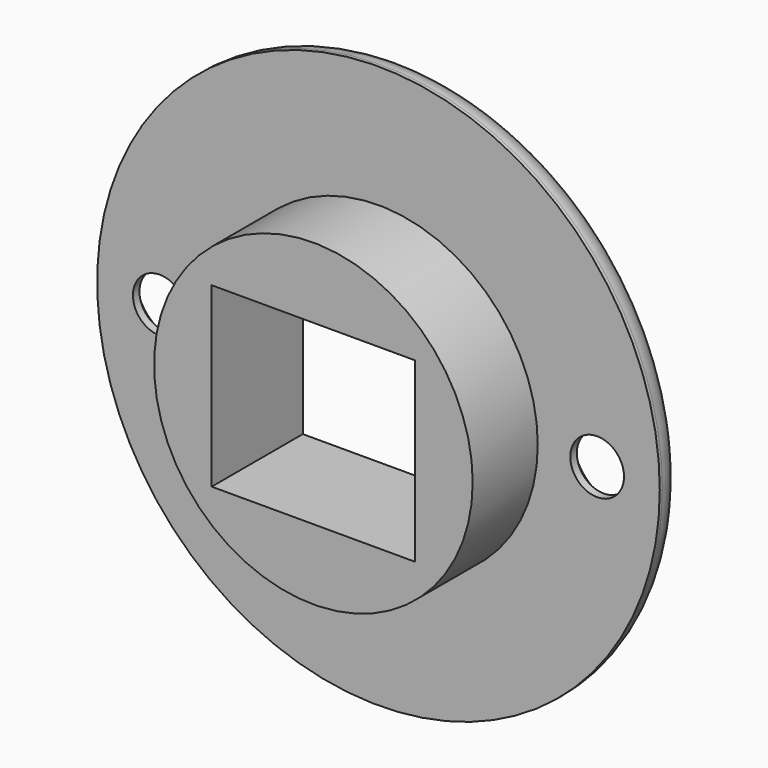
from build123d import *

# Parameters (mm, degrees)
F0_R     = 17.2924664606
F0_R_2   = 1.65
F0_R_3   = 9.7924664606
F1_DEPTH = 2
F2_DEPTH = 5
F3_SIZE  = 1.5


# Not quite as in the source:
# - a fillet or chamfer that OpenCascade refuses, or shapes differently, is made with other operations: its cross-section is extruded or revolved along the edge and cut away or added


with BuildPart() as f1:
    # F0 (on Front) → F1 (new body)
    with BuildSketch(Plane.XZ):
        Circle(F0_R)
        with Locations((-13.4424664606, 0)):
            Circle(F0_R_2, mode=Mode.SUBTRACT)
        Circle(F0_R_3, mode=Mode.SUBTRACT)
        with Locations((13.4424664606, 0)):
            Circle(F0_R_2, mode=Mode.SUBTRACT)
        Circle(F0_R_3)
        with BuildLine():
            ThreePointArc((8.2924664606, 0), (7.7650793743, -2.9100759974), (6.25, -5.45))
            ThreePointArc((6.25, -5.45), (0, -8.2924664606), (-6.25, -5.45))
            ThreePointArc((-6.25, -5.45), (-8.2924664606, 0), (-6.25, 5.45))
            ThreePointArc((-6.25, 5.45), (0, 8.2924664606), (6.25, 5.45))
            ThreePointArc((6.25, 5.45), (7.7650793743, 2.9100759974), (8.2924664606, 0))
        make_face(mode=Mode.SUBTRACT)
        with BuildLine():
            ThreePointArc((-6.25, 5.45), (-8.2924664606, 0), (-6.25, -5.45))
            Line((-6.25, -5.45), (-6.25, 5.45))
        make_face()
        with BuildLine():
            Line((-6.25, 5.45), (6.25, 5.45))
            ThreePointArc((6.25, 5.45), (0, 8.2924664606), (-6.25, 5.45))
        make_face()
        with BuildLine():
            Line((6.25, 5.45), (6.25, -5.45))
            ThreePointArc((6.25, -5.45), (7.7650793743, -2.9100759974), (8.2924664606, 0))
            ThreePointArc((8.2924664606, 0), (7.7650793743, 2.9100759974), (6.25, 5.45))
        make_face()
        with BuildLine():
            ThreePointArc((-6.25, -5.45), (0, -8.2924664606), (6.25, -5.45))
            Line((6.25, -5.45), (-6.25, -5.45))
        make_face()
    extrude(amount=-F1_DEPTH)

    # F0 (on Front) → F2 (join)
    with BuildSketch(Plane.XZ):
        Circle(F0_R_3)
        with BuildLine():
            ThreePointArc((8.2924664606, 0), (7.7650793743, -2.9100759974), (6.25, -5.45))
            ThreePointArc((6.25, -5.45), (0, -8.2924664606), (-6.25, -5.45))
            ThreePointArc((-6.25, -5.45), (-8.2924664606, 0), (-6.25, 5.45))
            ThreePointArc((-6.25, 5.45), (0, 8.2924664606), (6.25, 5.45))
            ThreePointArc((6.25, 5.45), (7.7650793743, 2.9100759974), (8.2924664606, 0))
        make_face(mode=Mode.SUBTRACT)
        with BuildLine():
            ThreePointArc((-6.25, 5.45), (-8.2924664606, 0), (-6.25, -5.45))
            Line((-6.25, -5.45), (-6.25, 5.45))
        make_face()
        with BuildLine():
            Line((-6.25, 5.45), (6.25, 5.45))
            ThreePointArc((6.25, 5.45), (0, 8.2924664606), (-6.25, 5.45))
        make_face()
        with BuildLine():
            Line((6.25, 5.45), (6.25, -5.45))
            ThreePointArc((6.25, -5.45), (7.7650793743, -2.9100759974), (8.2924664606, 0))
            ThreePointArc((8.2924664606, 0), (7.7650793743, 2.9100759974), (6.25, 5.45))
        make_face()
        with BuildLine():
            ThreePointArc((-6.25, -5.45), (0, -8.2924664606), (6.25, -5.45))
            Line((6.25, -5.45), (-6.25, -5.45))
        make_face()
    extrude(amount=F2_DEPTH)

    # F3
    f3_edges = [f1.edges().sort_by_distance(p)[0] for p in [
        (11.792466, 2, 0),
        (-15.092466, 2, 0),
    ]]
    chamfer(f3_edges, length=F3_SIZE)

    # F4: fillet of radius 1.8 on 1 edges, made by hand

    # F4_s1 → F4_t2 (revolve, cut)
    with BuildSketch(Plane.XY):
        with BuildLine():
            ThreePointArc((15.4924664606, 2), (16.7652586667, 1.4727922061), (17.2924664606, 0.2))
            Line((17.2924664606, 0.2), (17.2924664606, 2))
            Line((17.2924664606, 2), (15.4924664606, 2))
        make_face()
    revolve(axis=Axis((0, 2, 0), (0, -1, 0)), mode=Mode.SUBTRACT)


solid = f1.part
